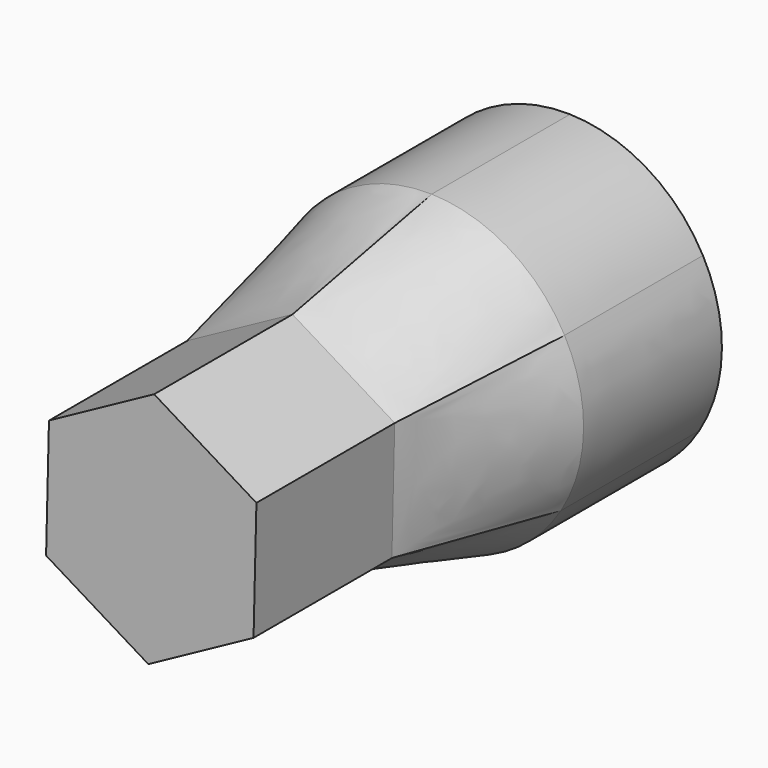
from build123d import *

# Parameters (mm, degrees)
F4_DEPTH = 5
F5_DEPTH = 5
F7_DEPTH = 5


# Not quite as in the source:
# - the arcs of a loft's sections are written as splines that run evenly, so that the points pair up as in the source's solid


with BuildPart() as f3:
    # F0 (on Front) → F3 section 0
    with BuildSketch(Plane.XZ):
        with BuildLine():
            add(Edge.make_bspline(
                [(3.8418426736, -2.3431271565), (4.1144778981, -1.8961084632), (4.3082439854, -1.4011386227), (4.5148518075, -0.3745248107), (4.5276427142, 0.1568666009), (4.3706679569, 1.1922320614), (4.2009409107, 1.6959513974), (3.9501289786, 2.1555697744)],
                knots=[0, 0, 0, 0, 0.3333333333, 0.3333333333, 0.6666666667, 0.6666666667, 1, 1, 1, 1], degree=3))
            add(Edge.make_bspline(
                [(3.9501289786, 2.1555697744), (3.6993170465, 2.6151881514), (3.3675436342, 3.0304794257), (2.5817739042, 3.7227139543), (2.1279708957, 3.9994869102), (1.1528307261, 4.3812255129), (0.6317334617, 4.4860972472), (0.1082863051, 4.4986969309)],
                knots=[0, 0, 0, 0, 0.3333333333, 0.3333333333, 0.6666666667, 0.6666666667, 1, 1, 1, 1], degree=3))
            add(Edge.make_bspline(
                [(0.1082863051, 4.4986969309), (-0.4151608516, 4.5112966146), (-0.9407003512, 4.4316180484), (-1.9330779034, 4.097238765), (-2.3996718185, 3.8426203093), (-3.2178372309, 3.1889934515), (-3.5692074491, 2.7901458498), (-3.8418426736, 2.3431271565)],
                knots=[0, 0, 0, 0, 0.3333333333, 0.3333333333, 0.6666666667, 0.6666666667, 1, 1, 1, 1], degree=3))
            add(Edge.make_bspline(
                [(-3.8418426736, 2.3431271565), (-4.1144778981, 1.8961084632), (-4.3082439854, 1.4011386227), (-4.5148518075, 0.3745248107), (-4.5276427142, -0.1568666009), (-4.3706679569, -1.1922320614), (-4.2009409107, -1.6959513974), (-3.9501289786, -2.1555697744)],
                knots=[0, 0, 0, 0, 0.3333333333, 0.3333333333, 0.6666666667, 0.6666666667, 1, 1, 1, 1], degree=3))
            add(Edge.make_bspline(
                [(-3.9501289786, -2.1555697744), (-3.6993170465, -2.6151881514), (-3.3675436342, -3.0304794257), (-2.5817739042, -3.7227139543), (-2.1279708957, -3.9994869102), (-1.1528307261, -4.3812255129), (-0.6317334617, -4.4860972472), (-0.1082863051, -4.4986969309)],
                knots=[0, 0, 0, 0, 0.3333333333, 0.3333333333, 0.6666666667, 0.6666666667, 1, 1, 1, 1], degree=3))
            add(Edge.make_bspline(
                [(-0.1082863051, -4.4986969309), (0.4151608516, -4.5112966146), (0.9407003512, -4.4316180484), (1.9330779034, -4.097238765), (2.3996718185, -3.8426203093), (3.2178372309, -3.1889934515), (3.5692074491, -2.7901458498), (3.8418426736, -2.3431271565)],
                knots=[0, 0, 0, 0, 0.3333333333, 0.3333333333, 0.6666666667, 0.6666666667, 1, 1, 1, 1], degree=3))
        make_face()
    # F2 (on offset) → F3 section 1
    with BuildSketch(Plane.XZ.offset(5)):
        Polygon((2.957451869, -1.8037401261), (3.0408107055, 1.659358386), (0.0833588365, 3.4630985121), (-2.957451869, 1.8037401261), (-3.0408107055, -1.659358386), (-0.0833588365, -3.4630985121), align=None)
    loft(ruled=True)

    # F4 (add): a face of the model
    f4_faces = [f3.faces().sort_by_distance(p)[0] for p in [
        (0, 0, 0),
    ]]
    extrude(f4_faces, amount=F4_DEPTH)

    # F5 (add): a face of the model
    f5_faces = [f3.faces().sort_by_distance(p)[0] for p in [
        (0, -5, 0),
    ]]
    extrude(f5_faces, amount=F5_DEPTH)

    # F6 (on Front) → F7 (cut)
    with BuildSketch(Plane.XZ):
        with BuildLine():
            ThreePointArc((1.5811388301, -2.25), (2.4403515918, -1.2677476518), (2.75, 0))
            ThreePointArc((2.75, 0), (-1.2677476518, 2.4403515918), (-1.5811388301, -2.25))
            Line((-1.5811388301, -2.25), (1.5811388301, -2.25))
        make_face()
    extrude(amount=-F7_DEPTH, mode=Mode.SUBTRACT)


solid = f3.part
